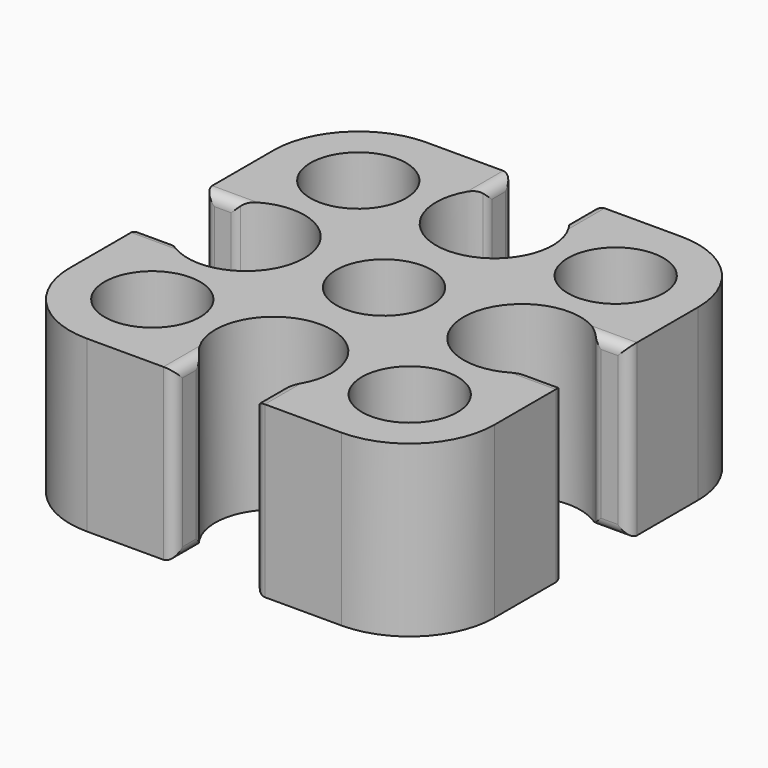
from build123d import *

# Parameters (mm, degrees)
F0_W             = 25.4
F0_H             = 25.4
F1_DEPTH         = 10.16
F2_R             = 3.4925
F3_DEPTH         = 25.4
F3_COPIES_COUNT  = 4
F5_DEPTH         = 25.4
F5_COPIES_COUNT  = 4
F7_R             = 2.8575
F8_DEPTH         = 25.4
F9_R             = 2.8575
F10_DEPTH        = 25.4
F10_COPIES_COUNT = 4
F11_R            = 5.08
F12_R            = 0.635


# Not quite as in the source:
# - a pattern or mirror of a feature is missing from the dataset's text; its kind, count and spacing are read off the source's solid


with BuildPart() as f1:
    # F0 (on Top) → F1 (new body)
    with BuildSketch(Plane.XY):
        Rectangle(F0_W, F0_H)
    extrude(amount=F1_DEPTH)

    # F2 (on face) → F3 (cut)
    with BuildSketch(Plane.XY.offset(10.16)):
        with Locations((0, -8.255)):
            Circle(F2_R)
    f3 = extrude(amount=-F3_DEPTH, mode=Mode.SUBTRACT)

    # F3_copies: F3 ×4 about axis
    f3_copies_axis = Axis((0, 0, 0), (0, 0, 1))
    for i in range(1, F3_COPIES_COUNT):
        add(f3.rotate(f3_copies_axis, i * 360 / F3_COPIES_COUNT), mode=Mode.SUBTRACT)

    # F4 (on face) → F5 (cut)
    with BuildSketch(Plane.XY.offset(10.16)):
        with BuildLine():
            Line((-2.3970724332, -10.795), (-2.3970724332, -12.7))
            Line((-2.3970724332, -12.7), (2.3970724332, -12.7))
            Line((2.3970724332, -12.7), (2.3970724332, -10.795))
            ThreePointArc((2.3970724332, -10.795), (0, -11.7475), (-2.3970724332, -10.795))
        make_face()
    f5 = extrude(amount=-F5_DEPTH, mode=Mode.SUBTRACT)

    # F5_copies: F5 ×4 about axis
    f5_copies_axis = Axis((0, 0, 0), (0, 0, 1))
    for i in range(1, F5_COPIES_COUNT):
        add(f5.rotate(f5_copies_axis, i * 360 / F5_COPIES_COUNT), mode=Mode.SUBTRACT)

    # F7 (on face) → F8 (cut)
    with BuildSketch(Plane.XY.offset(10.16)):
        Circle(F7_R)
    extrude(amount=-F8_DEPTH, mode=Mode.SUBTRACT)

    # F9 (on face) → F10 (cut)
    with BuildSketch(Plane.XY.offset(10.16)):
        with Locations((-7.7, 7.7)):
            Circle(F9_R)
    f10 = extrude(amount=-F10_DEPTH, mode=Mode.SUBTRACT)

    # F10_copies: F10 ×4 about axis
    f10_copies_axis = Axis((0, 0, 0), (0, 0, 1))
    for i in range(1, F10_COPIES_COUNT):
        add(f10.rotate(f10_copies_axis, i * 360 / F10_COPIES_COUNT), mode=Mode.SUBTRACT)

    # F11
    f11_edges = [f1.edges().sort_by_distance(p)[0] for p in [
        (-12.7, 12.7, 5.08),
        (-12.7, -12.7, 5.08),
        (12.7, -12.7, 5.08),
        (12.7, 12.7, 5.08),
    ]]
    fillet(f11_edges, radius=F11_R)

    # F12
    f12_edges = [f1.edges().sort_by_distance(p)[0] for p in [
        (2.397072, -11.7475, 10.16),
        (2.397072, -10.795, 5.08),
        (2.397072, -11.7475, 0),
        (2.397072, -12.7, 5.08),
        (-2.397072, -11.7475, 10.16),
        (-2.397072, -12.7, 5.08),
        (-2.397072, -11.7475, 0),
        (-2.397072, -10.795, 5.08),
        (11.7475, 2.397072, 0),
        (2.397072, 11.7475, 0),
        (11.7475, -2.397072, 0),
        (-2.397072, 11.7475, 0),
        (-11.7475, 2.397072, 0),
        (-11.7475, -2.397072, 0),
        (11.7475, 2.397072, 10.16),
        (2.397072, 11.7475, 10.16),
        (11.7475, -2.397072, 10.16),
        (-2.397072, 11.7475, 10.16),
        (-11.7475, 2.397072, 10.16),
        (-11.7475, -2.397072, 10.16),
        (12.7, 2.397072, 5.08),
        (10.795, 2.397072, 5.08),
        (2.397072, 12.7, 5.08),
        (10.795, -2.397072, 5.08),
        (2.397072, 10.795, 5.08),
        (12.7, -2.397072, 5.08),
        (-2.397072, 10.795, 5.08),
        (-2.397072, 12.7, 5.08),
        (-12.7, 2.397072, 5.08),
        (-10.795, 2.397072, 5.08),
        (-10.795, -2.397072, 5.08),
        (-12.7, -2.397072, 5.08),
    ]]
    fillet(f12_edges, radius=F12_R)


solid = f1.part
